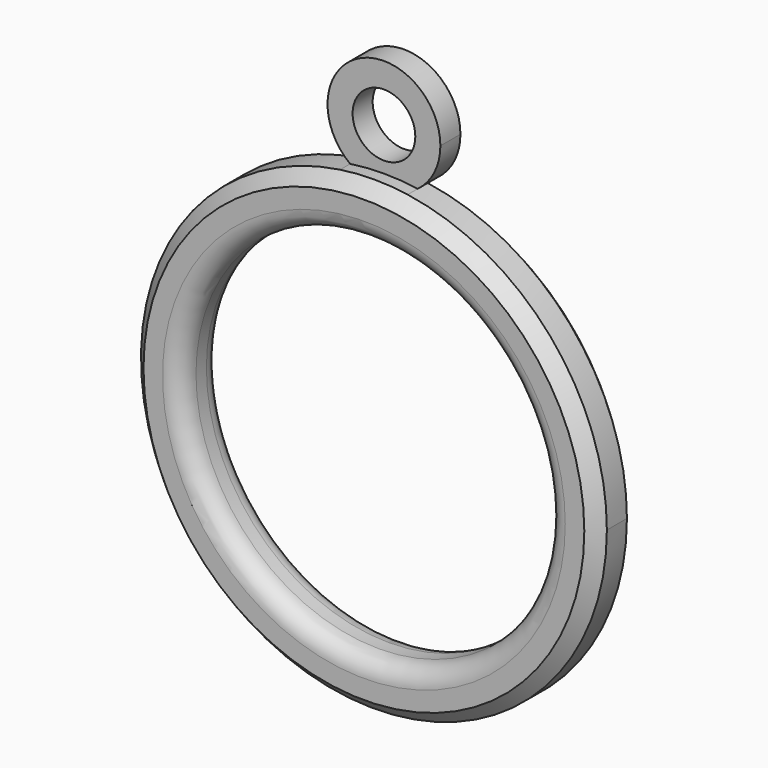
from build123d import *

# Parameters (mm, degrees)
F0_R         = 11.1125
F1_DEPTH     = 3.048
F0_R_2       = 1.905
F2_DEPTH     = 1.524
F3_R         = 1.1286206983
F4_T6_ANGLE  = 269.6278921261
F4_S7_R      = 3.429
F4_T8_DEPTH  = 22
F4_T12_ANGLE = 89.6035333551
F4_S13_R     = 3.429
F4_T14_DEPTH = 11


# Not quite as in the source:
# - a fillet or chamfer that OpenCascade refuses, or shapes differently, is made with other operations: its cross-section is extruded or revolved along the edge and cut away or added


with BuildPart() as f1:
    # F0 (on Front) → F1 (new body)
    with BuildSketch(Plane.XZ):
        with BuildLine():
            ThreePointArc((-2.05101646, 14.0111773856), (-9.2594908518, -10.713617009), (14.1605, 0))
            ThreePointArc((14.1605, 0), (10.713617009, 9.2594908518), (2.05101646, 14.0111773856))
            ThreePointArc((2.05101646, 14.0111773856), (0, 13.3301534555), (-2.05101646, 14.0111773856))
        make_face()
        Circle(F0_R, mode=Mode.SUBTRACT)
        with BuildLine():
            ThreePointArc((-2.05101646, 14.0111773856), (0, 13.3301534555), (2.05101646, 14.0111773856))
            ThreePointArc((2.05101646, 14.0111773856), (0, 14.1605), (-2.05101646, 14.0111773856))
        make_face()
    extrude(amount=F1_DEPTH)

    # F0 (on Front) → F2 (join)
    with BuildSketch(Plane.XZ):
        with BuildLine():
            ThreePointArc((-2.05101646, 14.0111773856), (0, 14.1605), (2.05101646, 14.0111773856))
            ThreePointArc((2.05101646, 14.0111773856), (3.065206065, 15.2220936716), (3.429, 16.7591534555))
            ThreePointArc((3.429, 16.7591534555), (-1.5370597839, 19.8243595205), (-2.05101646, 14.0111773856))
        make_face()
        with Locations((0, 16.7591534555)):
            Circle(F0_R_2, mode=Mode.SUBTRACT)
    extrude(amount=F2_DEPTH)

    # F3
    f3_edges = [f1.edges().sort_by_distance(p)[0] for p in [
        (11.1125, -1.524, 0),
        (-11.1125, 0, 0),
        (-11.1125, -3.048, 0),
    ]]
    fillet(f3_edges, radius=F3_R)

    # F4: chamfer of 0.762 on 2 edges, made by hand

    # F4_s1 → F4_t2 (revolve, cut)
    with BuildSketch(Plane.XY):
        Polygon((14.1605, -2.286), (13.3985, -3.048), (14.1605, -3.048), align=None)
    revolve(axis=Axis((0, -3.048, 0), (0, -1, 0)), mode=Mode.SUBTRACT)


with BuildPart() as f4_tool4:
    # F4_s5 → F4_t6 (revolve)
    with BuildSketch(Plane(origin=(0, 0, 0), x_dir=(0, 1, 0), z_dir=(0.9999789108, 0, 0.0064944619))):
        Polygon((0, 13.3985), (-0.762, 14.1605), (0, 14.1605), align=None)
    revolve(axis=Axis((0, 0, 0), (0, -1, 0)), revolution_arc=F4_T6_ANGLE)

    # F4_s7 → F4_t8 (cut, symmetric)
    with BuildSketch(Plane.XZ.offset(0.4)):
        with Locations((0, 16.7591534555)):
            Circle(F4_S7_R)
    extrude(amount=F4_T8_DEPTH, both=True, mode=Mode.SUBTRACT)


with BuildPart() as f1_1:
    add(f1.part)

    # F4_t3: cut F4_tool4
    add(f4_tool4.part, mode=Mode.SUBTRACT)


with BuildPart() as f4_tool10:
    # F4_s11 → F4_t12 (revolve)
    with BuildSketch(Plane.XY):
        Polygon((13.3985, 0), (14.1605, -0.762), (14.1605, 0), align=None)
    revolve(axis=Axis((0, 0, 0), (0, -1, 0)), revolution_arc=F4_T12_ANGLE)

    # F4_s13 → F4_t14 (cut, symmetric)
    with BuildSketch(Plane.XZ.offset(0.4)):
        with Locations((0, 16.7591534555)):
            Circle(F4_S13_R)
    extrude(amount=F4_T14_DEPTH, both=True, mode=Mode.SUBTRACT)


with BuildPart() as f1_2:
    add(f1_1.part)

    # F4_t9: cut F4_tool10
    add(f4_tool10.part, mode=Mode.SUBTRACT)


solid = f1_2.part
